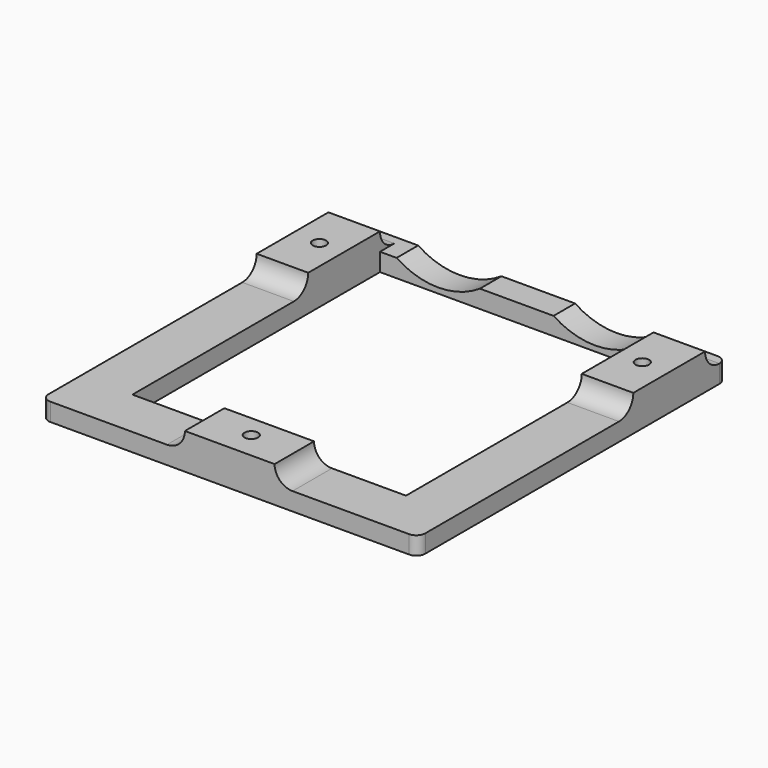
from build123d import *

# Parameters (mm, degrees)
F0_W     = 42
F0_H     = 43
F0_R     = 0.75
F0_W_2   = 30.5
F0_H_2   = 34.5
F1_DEPTH = 2
F2_W     = 5.75
F2_H     = 10
F2_R     = 0.75
F2_W_2   = 10
F2_H_2   = 5.5
F3_DEPTH = 2
F4_R     = 8.4
F5_DEPTH = 3
F6_R     = 1.99999
F7_R     = 1


# Not quite as in the source:
# - a fillet or chamfer is up to 0.001 mm smaller than in the source, because OpenCascade refuses the exact size


with BuildPart() as f1:
    # F0 (on Top) → F1 (new body)
    with BuildSketch(Plane.XY):
        with Locations((0, -18.5)):
            Rectangle(F0_W, F0_H)
        with Locations((0, -37)):
            Circle(F0_R, mode=Mode.SUBTRACT)
        with Locations((-18, -5)):
            Circle(F0_R, mode=Mode.SUBTRACT)
        with Locations((0, -17.25)):
            Rectangle(F0_W_2, F0_H_2, mode=Mode.SUBTRACT)
        with Locations((18, -5)):
            Circle(F0_R, mode=Mode.SUBTRACT)
    extrude(amount=F1_DEPTH)

    # F2 (on face) → F3 (join)
    with BuildSketch(Plane.XY.offset(2)):
        with Locations((-18.125, -5)):
            Rectangle(F2_W, F2_H)
        with Locations((-18, -5)):
            Circle(F2_R, mode=Mode.SUBTRACT)
        with Locations((18.125, -5)):
            Rectangle(F2_W, F2_H)
        with Locations((18, -5)):
            Circle(F2_R, mode=Mode.SUBTRACT)
        with Locations((0, -37.25)):
            Rectangle(F2_W_2, F2_H_2)
        with Locations((0, -37)):
            Circle(F2_R, mode=Mode.SUBTRACT)
    extrude(amount=F3_DEPTH)

    # F4 (on face) → F5 (cut, through all)
    with BuildSketch(Plane(origin=(0, 3, 0), x_dir=(-1, 0, 0), z_dir=(0, 1, 0))):
        with Locations((-8.75, 9)):
            Circle(F4_R)
        with Locations((8.75, 9)):
            Circle(F4_R)
    extrude(amount=-F5_DEPTH, mode=Mode.SUBTRACT)

    # F6 (radius 2 in the source; OpenCascade refuses exactly that, so slightly less here)
    f6_edges = [f1.edges().sort_by_distance(p)[0] for p in [
        (5, -37.25, 2),
        (18.125, -10, 2),
        (-18.125, -10, 2),
        (-5, -37.25, 2),
        (18.125, 0, 2),
        (-18.125, 0, 2),
    ]]
    fillet(f6_edges, radius=F6_R)

    # F7
    f7_edges = [f1.edges().sort_by_distance(p)[0] for p in [
        (-21, -40, 1),
        (-21, 3, 1),
        (21, -40, 1),
        (21, 3, 1),
    ]]
    fillet(f7_edges, radius=F7_R)


solid = f1.part
